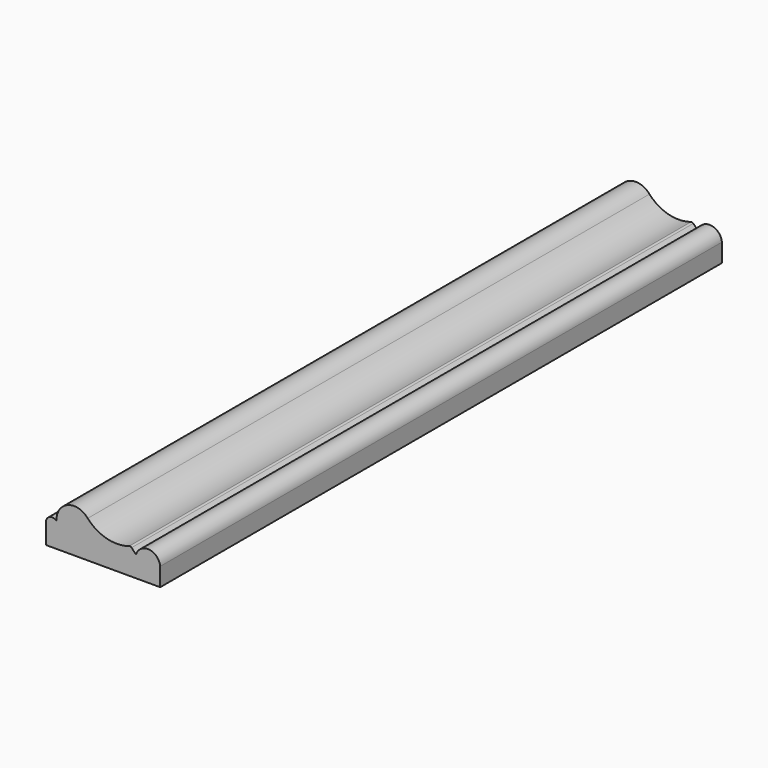
from build123d import *

# Parameters (mm, degrees)
F1_DEPTH = 152.4


# Not quite as in the source:
# - ends of sketch curves that miss each other by under 0.0002 mm in the source are joined


with BuildPart() as f1:
    # F0 (on Front) → F1 (new body)
    with BuildSketch(Plane.XZ):
        with BuildLine():
            Line((-12.3838716, -0.0228854), (-12.3838716, -4.7218854))
            Line((-12.3838716, -4.7218854), (12.383897, -4.7218854))
            Line((12.383897, -4.7218854), (12.383897, -0.7239254))
            ThreePointArc((12.383897, -0.7239254), (9.9901302454, 1.6896267796), (7.1382289827, -0.1602538356))
            Line((7.1382289827, -0.1602538356), (6.1675772, 0.81153))
            ThreePointArc((6.1675772, 0.81153), (5.9240303947, 0.9642906727), (5.6377868977, 0.9375583076))
            ThreePointArc((5.6377868977, 0.9375583076), (0.7948702497, 0.8064034512), (-3.3428712434, 3.3263562022))
            ThreePointArc((-3.3428712434, 3.3263562022), (-7.7001712998, 4.4538085328), (-10.1053789302, 0.6495786484))
            ThreePointArc((-10.1053789302, 0.6495786484), (-11.4361565644, 0.9623164645), (-12.3838716, -0.0228854))
        make_face()
    extrude(amount=F1_DEPTH)


solid = f1.part
